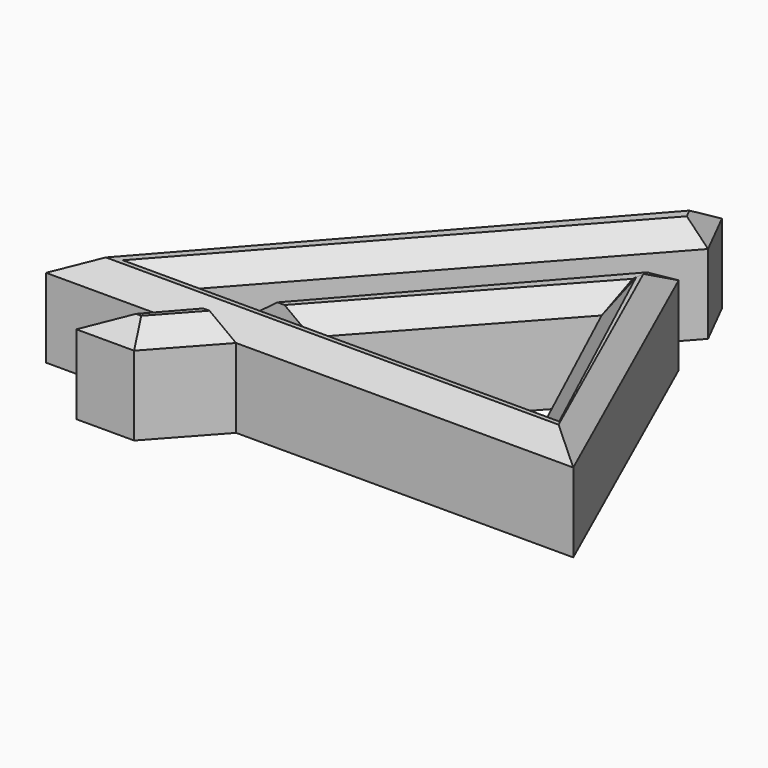
from build123d import *

# Parameters (mm, degrees)
F1_DEPTH  = 12.7
F2_DEPTH  = 12.7
F3_SIZE   = 2.54
F3_2_SIZE = 2.54
F3_3_SIZE = 2.54


with BuildPart() as f1:
    # F0 (on Top) → F1 (new body)
    with BuildSketch(Plane.XY):
        Polygon((-17.142418772, 38.3483767509), (-45.9020223429, 5.6663663127), (-38.1771805871, 5.6663663127), (-18.4063371271, 27.5632161647), align=None)
    extrude(amount=F1_DEPTH)

    # F3#2
    f3_2_edges = [f1.edges().sort_by_distance(p)[0] for p in [
        (-28.291759, 16.614791, 12.7),
        (-31.522221, 22.007372, 12.7),
    ]]
    chamfer(f3_2_edges, length=F3_2_SIZE)


with BuildPart() as f1b:
    # F0 (on Top) → F1, piece 2 (new body)
    with BuildSketch(Plane.XY):
        Polygon((-43.2933887226, 0), (-50.8883266324, 0), (-57.6514452696, -7.6855132356), (-50.2327010036, -7.6855132356), align=None)
    extrude(amount=F1_DEPTH)

    # F3#3
    f3_3_edges = [f1b.edges().sort_by_distance(p)[0] for p in [
        (-46.763045, -3.842757, 12.7),
        (-54.269886, -3.842757, 12.7),
        (-53.942073, -7.685513, 12.7),
    ]]
    chamfer(f3_3_edges, length=F3_3_SIZE)


with BuildPart() as f2:
    # F0 (on Top) → F2 (new body)
    with BuildSketch(Plane.XY):
        Polygon((0, 0), (-17.142418772, 38.3483767509), (-18.4063371271, 27.5632161647), (-8.2830116153, 5.6663663127), (-38.1771805871, 5.6663663127), (-43.2933887226, 0), align=None)
        Polygon((-38.1771805871, 5.6663663127), (-45.9020223429, 5.6663663127), (-50.8883266324, 0), (-43.2933887226, 0), align=None)
        Polygon((-54.6591710989, 5.6663663127), (-19.0966203809, 45.5031730235), (-22.1344456077, 51.5287555754), (-67.6876604557, 0), (-59.7175695002, 0), (-50.8883266324, 0), (-45.9020223429, 5.6663663127), align=None)
    extrude(amount=F2_DEPTH)

    # F3
    f3_edges = [f2.edges().sort_by_distance(p)[0] for p in [
        (-33.84383, 0, 12.7),
        (-31.471091, 5.666366, 12.7),
        (-13.344674, 16.614791, 12.7),
        (-8.571209, 19.174188, 12.7),
        (-44.911053, 25.764378, 12.7),
        (-36.877896, 25.58477, 12.7),
        (-20.615533, 48.515964, 12.7),
    ]]
    chamfer(f3_edges, length=F3_SIZE)


solid = Compound([f1.part, f1b.part, f2.part])
